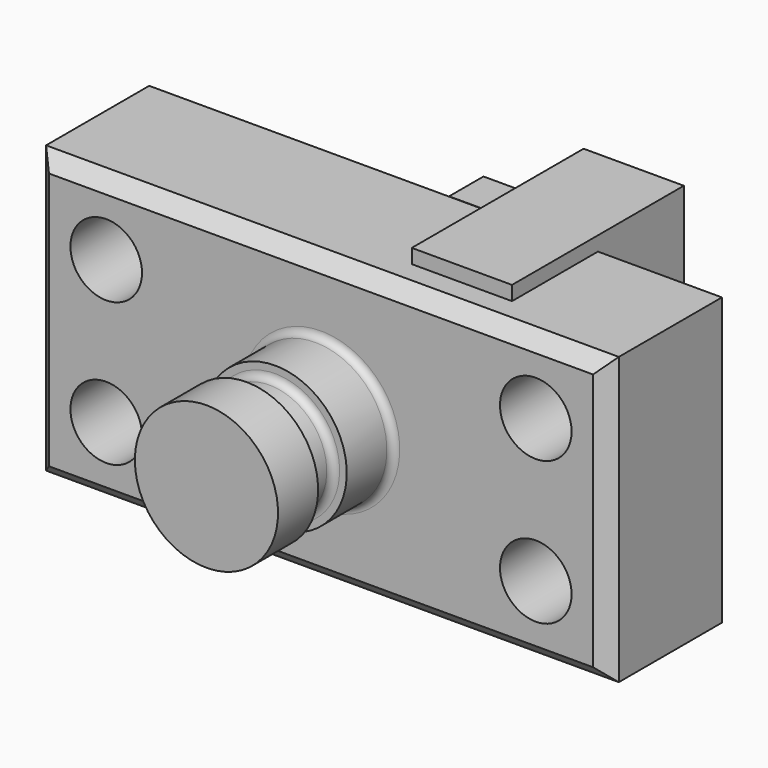
from build123d import *

# Parameters (mm, degrees)
F0_W      = 101.6
F0_H      = 50.8
F1_DEPTH  = 25.4
F2_R      = 6.35
F3_DEPTH  = 25.401
F4_W      = 12.7
F4_H      = 25.4
F6_W      = 5.7951804488
F6_H      = 6.35
F8_R      = 1.27
F9_SIZE   = 2.54
F10_W     = 57.15
F10_H     = 38.1
F11_DEPTH = 7.62
F12_W     = 17.78
F12_H     = 38.1
F13_DEPTH = 27.94
F14_W     = 17.78
F14_H     = 7.62
F15_DEPTH = 17.78


with BuildPart() as f1:
    # F0 (on Front) → F1 (new body)
    with BuildSketch(Plane.XZ):
        Rectangle(F0_W, F0_H)
    extrude(amount=F1_DEPTH)

    # F2 (on face) → F3 (cut, through all)
    with BuildSketch(Plane.XZ.offset(25.4)):
        with Locations((-38.1, 12.7)):
            Circle(F2_R)
        with Locations((-38.1, -12.7)):
            Circle(F2_R)
        with Locations((38.1, 12.7)):
            Circle(F2_R)
        with Locations((38.1, -12.7)):
            Circle(F2_R)
    extrude(amount=-F3_DEPTH, mode=Mode.SUBTRACT)

    # F4 (on Top) → F5 (revolve)
    with BuildSketch(Plane.XY):
        with Locations((-6.35, -38.1)):
            Rectangle(F4_W, F4_H)
    revolve(axis=Axis((0, -38.1, 0), (0, -1, 0)))

    # F6 (on Top) → F7 (revolve, cut)
    with BuildSketch(Plane.XY):
        with Locations((-13.0575902244, -38.735)):
            Rectangle(F6_W, F6_H)
    revolve(axis=Axis((0, -9.0271439403, 0), (0, -1, 0)), mode=Mode.SUBTRACT)

    # F8
    f8_edges = [f1.edges().sort_by_distance(p)[0] for p in [
        (12.7, -25.4, 0),
        (10.16, -41.91, 0),
        (10.16, -35.56, 0),
    ]]
    fillet(f8_edges, radius=F8_R)

    # F9
    f9_edges = [f1.edges().sort_by_distance(p)[0] for p in [
        (0, -25.4, -25.4),
        (-50.8, -25.4, 0),
        (0, -25.4, 25.4),
        (50.8, -25.4, 0),
    ]]
    chamfer(f9_edges, length=F9_SIZE)


with BuildPart() as f11:
    # F10 (on Top) → F11 (new body)
    with BuildSketch(Plane.XY):
        Rectangle(F10_W, F10_H)
    extrude(amount=F11_DEPTH)

    # F12 (on Top) → F13 (join)
    with BuildSketch(Plane.XY):
        with Locations((19.9131323025, 0)):
            Rectangle(F12_W, F12_H)
    extrude(amount=F13_DEPTH)

    # F14 (on Top) → F15 (join)
    with BuildSketch(Plane.XY):
        with Locations((2.094425433, 15.3110322082)):
            Rectangle(F14_W, F14_H)
        with Locations((1.9588155529, -15.1754241908)):
            Rectangle(F14_W, F14_H)
    extrude(amount=F15_DEPTH)


solid = Compound([f1.part, f11.part])
